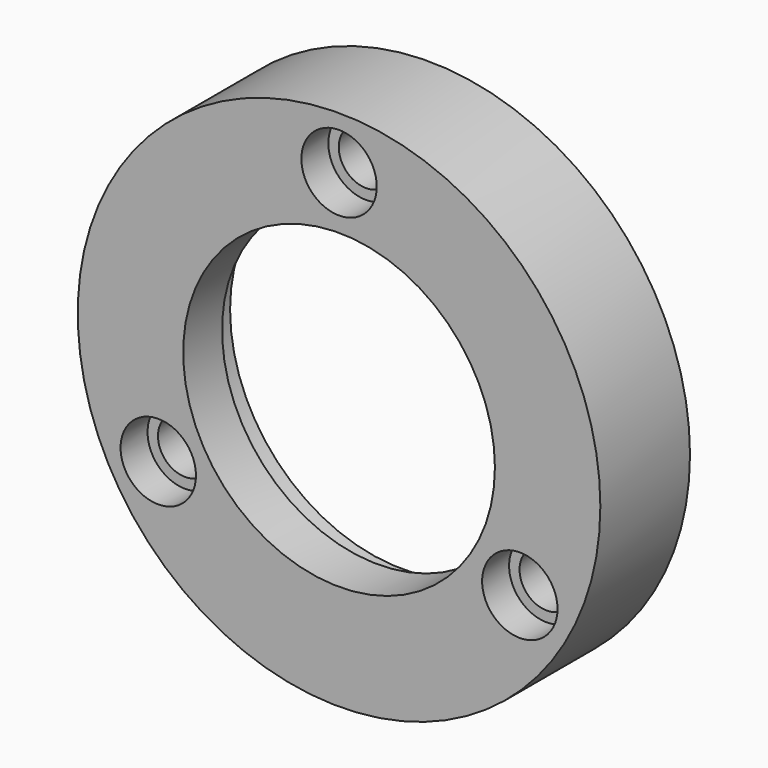
from build123d import *

# Parameters (mm, degrees)
F0_R            = 26.35
F0_R_2          = 15.7166947943
F1_DEPTH        = 11.3
F2_R            = 17.3887467131
F2_R_2          = 15.7166947943
F3_DEPTH        = 6.4
F4_R            = 24.35
F4_R_2          = 17.3887467131
F5_DEPTH        = 3.3
F6_R            = 3.8017714644
F6_R_2          = 2.75
F7_DEPTH        = 3.4
F7_COPIES_COUNT = 3
F8_DEPTH        = 10
F8_COPIES_COUNT = 3


# Not quite as in the source:
# - a feature of the source that left no trace in its solid (it failed there, or was rolled back) is left out
# - a pattern or mirror of a feature is missing from the dataset's text; its kind, count and spacing are read off the source's solid


with BuildPart() as f1:
    # F0 (on Front) → F1 (new body)
    with BuildSketch(Plane.XZ):
        Circle(F0_R)
        Circle(F0_R_2, mode=Mode.SUBTRACT)
    extrude(amount=F1_DEPTH)

    # F2 (on face) → F3 (cut)
    with BuildSketch(Plane(origin=(0, 0, 0), x_dir=(-1, 0, 0), z_dir=(0, 1, 0))):
        Circle(F2_R)
        Circle(F2_R_2, mode=Mode.SUBTRACT)
    extrude(amount=-F3_DEPTH, mode=Mode.SUBTRACT)

    # F4 (on face) → F5 (cut)
    with BuildSketch(Plane(origin=(0, 0, 0), x_dir=(-1, 0, 0), z_dir=(0, 1, 0))):
        Circle(F4_R)
        Circle(F4_R_2, mode=Mode.SUBTRACT)
    extrude(amount=-F5_DEPTH, mode=Mode.SUBTRACT)

    # F6 (on face) → F7 (cut)
    with BuildSketch(Plane.XZ.offset(11.3)):
        with Locations((0, 21.05)):
            Circle(F6_R)
        with Locations((0, 21.05)):
            Circle(F6_R_2, mode=Mode.SUBTRACT)
    f7 = extrude(amount=-F7_DEPTH, mode=Mode.SUBTRACT)

    # F7_copies: F7 ×3 about axis
    f7_copies_axis = Axis((0, 0, 0), (0, 1, 0))
    for i in range(1, F7_COPIES_COUNT):
        add(f7.rotate(f7_copies_axis, i * 360 / F7_COPIES_COUNT), mode=Mode.SUBTRACT)

    # F8 (cut): a face of the model
    f8_faces = [f1.faces().sort_by_distance(p)[0] for p in [
        (0, -11.3, 21.05),
    ]]
    f8 = extrude(f8_faces, amount=-F8_DEPTH, mode=Mode.SUBTRACT)

    # F8_copies: F8 ×3 about axis
    f8_copies_axis = Axis((0, 0, 0), (0, 1, 0))
    for i in range(1, F8_COPIES_COUNT):
        add(f8.rotate(f8_copies_axis, i * 360 / F8_COPIES_COUNT), mode=Mode.SUBTRACT)


solid = f1.part
